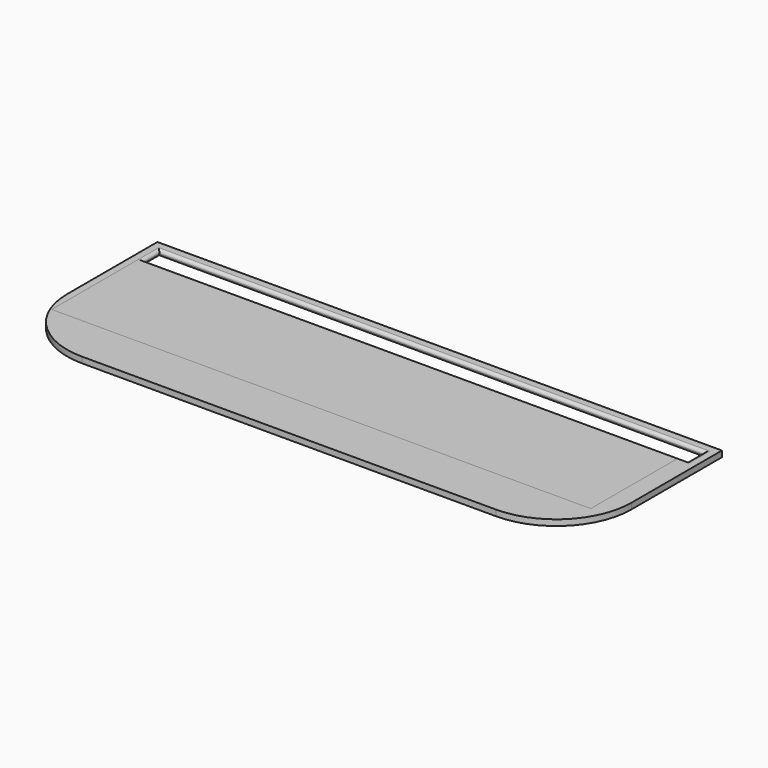
from build123d import *

# Parameters (mm, degrees)
F0_W         = 190.5
F0_H         = 63.5
F1_DEPTH     = 2
F2_W         = 183.896
F2_H         = 7.62
F3_DEPTH     = 25.4
F4_R         = 0.99999
F5_R         = 0.99999
F6_R         = 25.4
F7_TEXT_SIZE = 28.858512338
F8_DEPTH     = 2
F9_W         = 181.9221750228
F9_H         = 36.5569271355
F10_DEPTH    = 0.5
F11_W        = 177.9483407736
F11_H        = 26.1296071112
F12_DEPTH    = 0.5


# Not quite as in the source:
# - a fillet or chamfer is up to 0.001 mm smaller than in the source, because OpenCascade refuses the exact size
# - Text() gives the source's letters only with a copy of the font that has no kerning and outlines rounded to 1/6400 em; it was checked with that copy


with BuildPart() as f1:
    # F0 (on Top) → F1 (new body)
    with BuildSketch(Plane.XY):
        with Locations((1.791532172, 31.75)):
            Rectangle(F0_W, F0_H)
    extrude(amount=F1_DEPTH)

    # F2 (on face) → F3 (cut)
    with BuildSketch(Plane.XY.offset(2)):
        with Locations((1.791532172, 56.388)):
            Rectangle(F2_W, F2_H)
    extrude(amount=-F3_DEPTH, mode=Mode.SUBTRACT)

    # F4 (radius 1 in the source; OpenCascade refuses exactly that, so slightly less here)
    f4_edges = [f1.edges().sort_by_distance(p)[0] for p in [
        (1.791532, 60.198, 2),
        (1.791532, 60.198, 0),
    ]]
    fillet(f4_edges, radius=F4_R)

    # F5 (radius 1 in the source; OpenCascade refuses exactly that, so slightly less here)
    f5_edges = [f1.edges().sort_by_distance(p)[0] for p in [
        (93.739532, 56.388, 0),
        (93.739532, 56.388, 2),
        (-90.156468, 56.388, 2),
        (-90.156468, 56.388, 0),
    ]]
    fillet(f5_edges, radius=F5_R)

    # F6
    f6_edges = [f1.edges().sort_by_distance(p)[0] for p in [
        (-93.458468, 0, 1),
        (97.041532, 0, 1),
    ]]
    fillet(f6_edges, radius=F6_R)

    # F7 (on face) → F8 (cut)
    with BuildSketch(Plane.XY.offset(2)):
        with Locations((-87.108467828, 17.78)):
            Text('Shane Knott', F7_TEXT_SIZE, font='Open Sans', font_style=FontStyle.BOLD, text_align=(TextAlign.LEFT, TextAlign.BOTTOM))
    extrude(amount=-F8_DEPTH, mode=Mode.SUBTRACT)


with BuildPart() as f10:
    # F9 (on face) → F10 (new body)
    with BuildSketch(Plane.XY.offset(2)):
        with Locations((-0.1953803166, 34.2995364323)):
            Rectangle(F9_W, F9_H)
    extrude(amount=-F10_DEPTH)


with BuildPart() as f12:
    # F11 (on face) → F12 (new body)
    with BuildSketch(Plane(origin=(0, 0, 0), x_dir=(1, 0, 0), z_dir=(0, 0, -1))):
        with Locations((1.410074532, -28.8951490074)):
            Rectangle(F11_W, F11_H)
    extrude(amount=-F12_DEPTH)


solid = Compound([f1.part, f10.part, f12.part])
